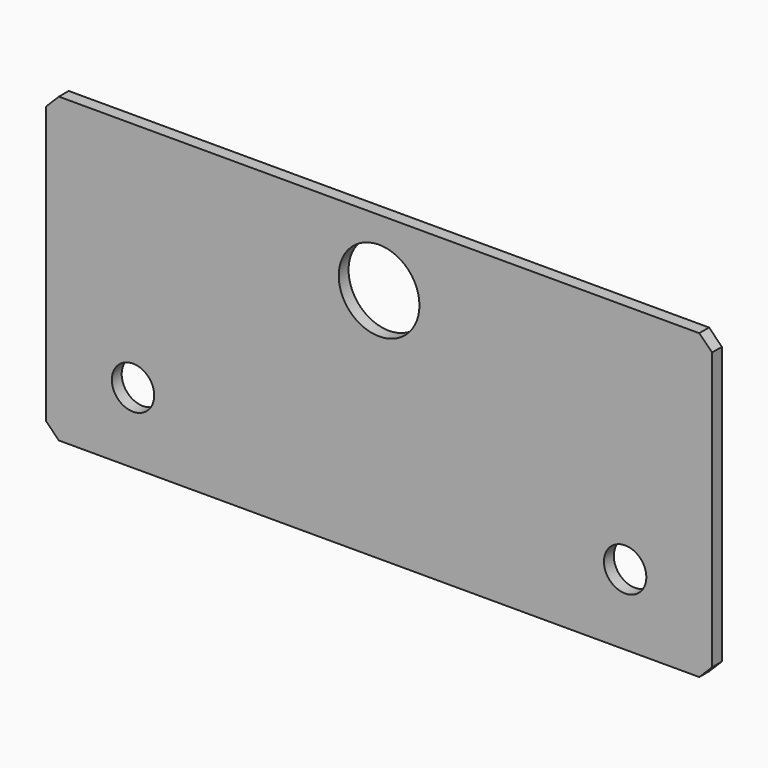
from build123d import *

# Parameters (mm, degrees)
F0_W     = 165
F0_H     = 75
F1_DEPTH = 3.048
F2_R     = 5.25
F3_DEPTH = 3.048
F4_R     = 10
F5_DEPTH = 3.048
F6_SIZE  = 3.175


# Not quite as in the source:
# - a pattern or mirror of a feature is missing from the dataset's text; its kind, count and spacing are read off the source's solid


with BuildPart() as f1:
    # F0 (on Front) → F1 (new body)
    with BuildSketch(Plane.XZ):
        with Locations((0, 37.5)):
            Rectangle(F0_W, F0_H)
    extrude(amount=F1_DEPTH)

    # F2 (on face) → F3 (cut)
    with BuildSketch(Plane.XZ.offset(3.048)):
        with Locations((-60.96, 17.5)):
            Circle(F2_R)
    f3 = extrude(amount=-F3_DEPTH, mode=Mode.SUBTRACT)

    # F3_copies: F3 across plane
    add(f3.mirror(Plane(origin=(0, 0, 0), x_dir=(0, 0, 1), z_dir=(1, 0, 0))), mode=Mode.SUBTRACT)

    # F4 (on face) → F5 (cut)
    with BuildSketch(Plane.XZ.offset(3.048)):
        with Locations((0, 58.5)):
            Circle(F4_R)
    extrude(amount=-F5_DEPTH, mode=Mode.SUBTRACT)

    # F6
    f6_edges = [f1.edges().sort_by_distance(p)[0] for p in [
        (-82.5, -1.524, 75),
        (-82.5, -1.524, 0),
        (82.5, -1.524, 0),
        (82.5, -1.524, 75),
    ]]
    chamfer(f6_edges, length=F6_SIZE)


solid = f1.part
